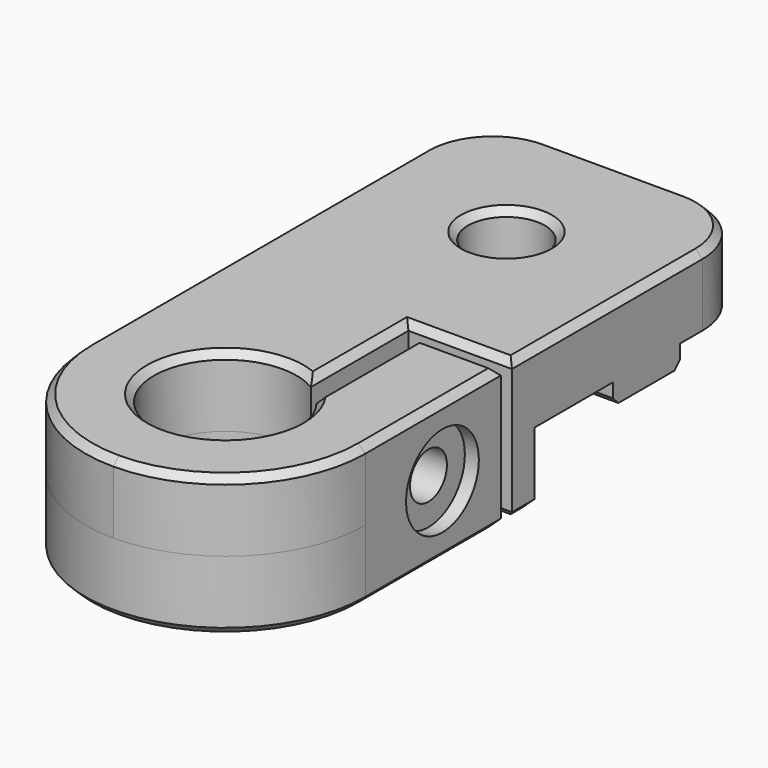
from build123d import *

# Parameters (mm, degrees)
F1_DEPTH       = 5
F3_DEPTH       = 5
F5_D           = 3.3
F5_DEPTH       = 26
F5_CBORE_D     = 6.5
F5_CBORE_DEPTH = 1
F5_TIP         = 0.9914200214
F7_DEPTH       = 3
F9_DEPTH       = 1.5
F10_D          = 5.5
F10_DEPTH      = 26
F10_TIP        = 1.6523667023
F11_SIZE       = 0.5
F13_R          = 5
F14_SIZE       = 0.5


with BuildPart() as f1:
    # F0 (on Top) → F1 (new body)
    with BuildSketch(Plane.XY):
        with BuildLine():
            Line((10, 0), (-10, 0))
            Line((-10, 0), (-10, -35.1))
            ThreePointArc((-10, -35.1), (-7.0710678119, -42.1710678119), (0, -45.1))
            ThreePointArc((0, -45.1), (7.0710678119, -42.1710678119), (10, -35.1))
            Line((10, -35.1), (10, -23))
            Line((10, -23), (4.1, -23))
            Line((4.1, -23), (4.1, -32.0668498224))
            ThreePointArc((4.1, -32.0668498224), (-3.4177556675, -38.8853594542), (2.6, -30.7125178063))
            Line((2.6, -30.7125178063), (2.6, -22))
            Line((2.6, -22), (10, -22))
            Line((10, -22), (10, 0))
        make_face()
    extrude(amount=F1_DEPTH)

    # F2 (on face) → F3 (join)
    with BuildSketch(Plane(origin=(0, 0, 0), x_dir=(1, 0, 0), z_dir=(0, 0, -1))):
        with BuildLine():
            Line((-10, 35.1), (-10, 20))
            Line((-10, 20), (10, 20))
            Line((10, 20), (10, 22))
            Line((10, 22), (2.6, 22))
            Line((2.6, 22), (2.6, 30.7125178063))
            ThreePointArc((2.6, 30.7125178063), (-3.4177556675, 38.8853594542), (4.1, 32.0668498224))
            Line((4.1, 32.0668498224), (4.1, 23))
            Line((4.1, 23), (10, 23))
            Line((10, 23), (10, 35.1))
            ThreePointArc((10, 35.1), (0, 45.1), (-10, 35.1))
        make_face()
    extrude(amount=F3_DEPTH)

    # F5
    with Locations(Plane.YZ.offset(10)):
        with Locations((-28.2125178063, 0)):
            CounterBoreHole(F5_D / 2, F5_CBORE_D / 2, F5_CBORE_DEPTH, depth=F5_DEPTH)
            with Locations((0, 0, -(F5_DEPTH + F5_TIP / 2))):  # 118° drill point
                Cone(0, F5_D / 2, F5_TIP, mode=Mode.SUBTRACT)

    # F6 (on face) → F7 (cut)
    with BuildSketch(Plane(origin=(-10, 0, 0), x_dir=(0, -1, 0), z_dir=(-1, 0, 0))):
        with BuildLine():
            Line((24.9216212719, 0), (26.5670695391, -2.85))
            Line((26.5670695391, -2.85), (29.8579660735, -2.85))
            Line((29.8579660735, -2.85), (31.5034143407, 0))
            Line((31.5034143407, 0), (29.8625178063, 0))
            ThreePointArc((29.8625178063, 0), (28.2125178063, -1.65), (26.5625178063, 0))
            Line((26.5625178063, 0), (24.9216212719, 0))
        make_face()
        with BuildLine():
            Line((26.5670695391, 2.85), (24.9216212719, 0))
            Line((24.9216212719, 0), (26.5625178063, 0))
            ThreePointArc((26.5625178063, 0), (28.2125178063, 1.65), (29.8625178063, 0))
            Line((29.8625178063, 0), (31.5034143407, 0))
            Line((31.5034143407, 0), (29.8579660735, 2.85))
            Line((29.8579660735, 2.85), (26.5670695391, 2.85))
        make_face()
    extrude(amount=-F7_DEPTH, mode=Mode.SUBTRACT)

    # F8 (on face) → F9 (join)
    with BuildSketch(Plane(origin=(0, 0, 0), x_dir=(1, 0, 0), z_dir=(0, 0, -1))):
        with BuildLine():
            ThreePointArc((-4.6097722286, 7), (-5.5, 10), (-4.6097722286, 13))
            Line((-4.6097722286, 13), (-10, 13))
            Line((-10, 13), (-10, 7))
            Line((-10, 7), (-4.6097722286, 7))
        make_face()
        with BuildLine():
            Line((10, 7), (10, 13))
            Line((10, 13), (4.6097722286, 13))
            ThreePointArc((4.6097722286, 13), (5.5, 10), (4.6097722286, 7))
            Line((4.6097722286, 7), (10, 7))
        make_face()
    extrude(amount=F9_DEPTH)

    # F10
    with Locations(Plane(origin=(0, 0, 0), x_dir=(1, 0, 0), z_dir=(0, 0, -1))):
        with Locations((0, 10)):
            Hole(F10_D / 2, depth=F10_DEPTH)
            with Locations((0, 0, -(F10_DEPTH + F10_TIP / 2))):  # 118° drill point
                Cone(0, F10_D / 2, F10_TIP, mode=Mode.SUBTRACT)

    # F11
    f11_edges = [f1.edges().sort_by_distance(p)[0] for p in [
        (-7.304886, -7, -1.5),
        (-7.304886, -13, -1.5),
        (7.304886, -13, -1.5),
        (7.304886, -7, -1.5),
    ]]
    chamfer(f11_edges, length=F11_SIZE)

    # F13
    f13_edges = [f1.edges().sort_by_distance(p)[0] for p in [
        (10, 0, 2.5),
        (-10, 0, 2.5),
    ]]
    fillet(f13_edges, radius=F13_R)

    # F14
    f14_edges = [f1.edges().sort_by_distance(p)[0] for p in [
        (10, -13.5, 5),
        (8.535534, -1.464466, 5),
        (6.3, -22, 5),
        (0, 0, 5),
        (2.6, -26.356259, 5),
        (-8.535534, -1.464466, 5),
        (-3.417756, -38.885359, 5),
        (-10, -20.05, 5),
        (4.1, -27.533425, 5),
        (0, -45.1, 5),
        (7.05, -23, 5),
        (10, -29.05, 5),
        (-2.75, -10, 5),
        (0, -45.1, -5),
        (-10, -27.55, -5),
        (0, -20, -5),
        (10, -21, -5),
        (6.3, -22, -5),
        (2.6, -26.356259, -5),
        (-3.417756, -38.885359, -5),
        (4.1, -27.533425, -5),
        (7.05, -23, -5),
        (10, -29.05, -5),
    ]]
    chamfer(f14_edges, length=F14_SIZE)


solid = f1.part
